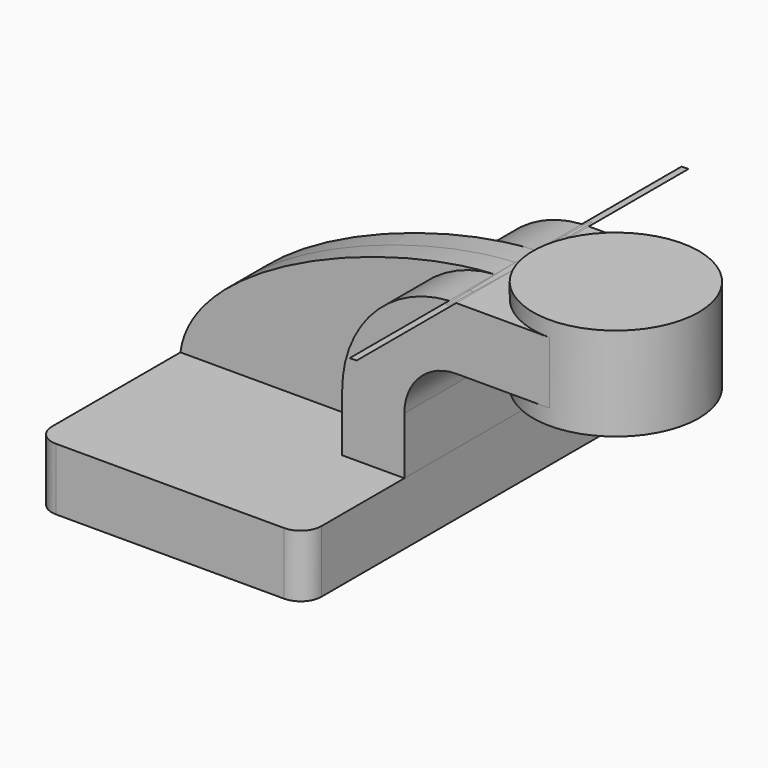
from build123d import *

# Parameters (mm, degrees)
F1_DEPTH = 63.5
F0_W     = 25.4
F0_H     = 19.0500000095
F2_DEPTH = 25.4
F3_DEPTH = 7.9375
F5_R     = 6.35


with BuildPart() as f1:
    # F0 (on Front) → F1 (new body, symmetric)
    with BuildSketch(Plane.XZ):
        with BuildLine():
            ThreePointArc((57.15, 61.9252000095), (56.0706314791, 61.9085169067), (54.9922941517, 61.8584835368))
            add(Edge.make_bspline(
                [(54.9922941517, 61.8584835368), (55.7230926251, 61.8907108689), (56.4425898793, 61.9130055057), (57.15, 61.9252000095)],
                knots=[109.1637569367, 109.1637569367, 109.1637569367, 109.1637569367, 111.504536168, 111.504536168, 111.504536168, 111.504536168], degree=3))
        make_face()
    extrude(amount=F1_DEPTH, both=True)


with BuildPart() as f1b:
    # F0 (on Front) → F1, piece 2 (new body, symmetric)
    with BuildSketch(Plane.XZ):
        Polygon((-41.275, -9.525), (41.275, -9.525), (41.275, 9.525), (22.2249999905, 9.525), (-41.275, 9.525), align=None)
    extrude(amount=F1_DEPTH, both=True)

    # F5
    f5_edges = [f1b.edges().sort_by_distance(p)[0] for p in [
        (41.275, -63.5, 0),
        (41.275, 63.5, 0),
        (-41.275, 63.5, 0),
        (-41.275, -63.5, 0),
    ]]
    fillet(f5_edges, radius=F5_R)


with BuildPart() as f2:
    # F0 (on Front) → F2 (new body, symmetric)
    with BuildSketch(Plane.XZ):
        with BuildLine():
            Line((22.2249999905, 9.525), (41.275, 9.525))
            Line((41.275, 9.525), (41.275, 27.0002))
            ThreePointArc((41.275, 27.0002), (45.9246798487, 38.2255201513), (57.15, 42.8752))
            Line((57.15, 42.8752), (60.325, 42.8752))
            Line((60.325, 42.8752), (60.325, 61.9252000095))
            Line((60.325, 61.9252000095), (57.15, 61.9252000095))
            add(Edge.make_bspline(
                [(54.9922941517, 61.8584835368), (55.7230926251, 61.8907108689), (56.4425898793, 61.9130055057), (57.15, 61.9252000095)],
                knots=[109.1637569367, 109.1637569367, 109.1637569367, 109.1637569367, 111.504536168, 111.504536168, 111.504536168, 111.504536168], degree=3))
            ThreePointArc((54.9922941517, 61.8584835368), (31.702863595, 50.920878804), (22.2249999905, 27.0002))
            Line((22.2249999905, 27.0002), (22.2249999905, 9.525))
        make_face()
        with Locations((73.025, 52.4002000047)):
            Rectangle(F0_W, F0_H)
    extrude(amount=F2_DEPTH, both=True)

    # F0 (on Front) → F4 (revolve)
    with BuildSketch(Plane.XZ):
        Polygon((85.725, 61.9252000095), (85.725, 42.8752), (85.725, 38.1), (111.125, 38.1), (111.125, 66.675), (85.725, 66.675), align=None)
    revolve(axis=Axis((85.725, 0, 52.3875), (0, 0, 1)))


with BuildPart() as f3:
    # F0 (on Front) → F3 (new body, symmetric)
    with BuildSketch(Plane.XZ):
        with BuildLine():
            add(Edge.make_bspline(
                [(-41.275, 9.525), (-37.7490644721, 37.2501413938), (20.9110335802, 60.3555410121), (54.9922941517, 61.8584835368)],
                knots=[0, 0, 0, 0, 109.1637569367, 109.1637569367, 109.1637569367, 109.1637569367], degree=3))
            Line((-41.275, 9.525), (22.2249999905, 9.525))
            Line((22.2249999905, 9.525), (22.2249999905, 27.0002))
            ThreePointArc((22.2249999905, 27.0002), (31.702863595, 50.920878804), (54.9922941517, 61.8584835368))
        make_face()
    extrude(amount=F3_DEPTH, both=True)


solid = Compound([f1.part, f1b.part, f2.part, f3.part])
